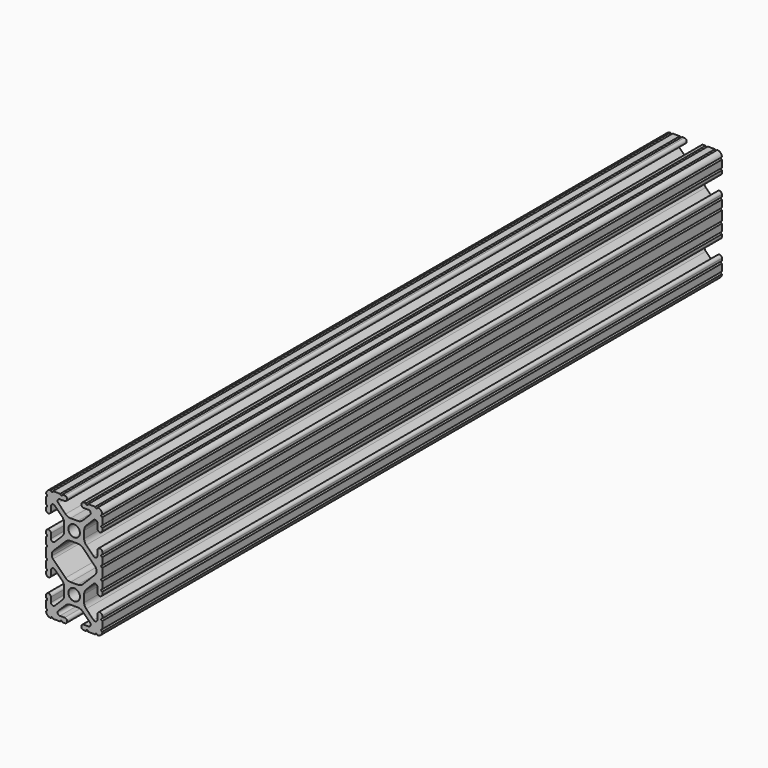
from build123d import *

# Parameters (mm, degrees)
F1_DEPTH = 350


# Not quite as in the source:
# - ends of sketch curves that miss each other by under 0.0002 mm in the source are joined


with BuildPart() as f1:
    # F0 (on Front) → F1 (new body)
    with BuildSketch(Plane.XZ):
        with BuildLine():
            ThreePointArc((-12.6999998568, 23.2791116031), (-12.1919492, 22.76475), (-12.6999998568, 22.2503883969))
            Line((-12.6999998568, 22.2503883969), (-12.7, 19.0246))
            ThreePointArc((-12.7, 19.0246), (-12.192, 18.5166), (-12.7, 18.0086))
            Line((-12.7, 18.0086), (-12.7, 17.0023028))
            ThreePointArc((-12.7, 17.0023028), (-11.5951, 15.8974028), (-10.4902, 17.0023028))
            Line((-10.4902, 17.0023028), (-10.4902, 19.1747902))
            ThreePointArc((-10.4902, 19.1747902), (-9.8630063673, 20.113451805), (-8.7557795103, 19.8932106897))
            Line((-8.7557795103, 19.8932106897), (-5.4384448, 16.5758622))
            ThreePointArc((-5.4384448, 16.5758622), (-4.7501824843, 15.5458268978), (-4.5085, 14.330807))
            Line((-4.5085, 14.330807), (-4.5085, 11.069193))
            ThreePointArc((-4.5085, 11.069193), (-4.7501824843, 9.8541731022), (-5.4384359697, 8.8241289697))
            Line((-5.4384359697, 8.8241289697), (-8.7557864, 5.5067962))
            ThreePointArc((-8.7557864, 5.5067962), (-9.8630063673, 5.286548195), (-10.4902, 6.2252098))
            Line((-10.4902, 6.2252098), (-10.4902, 8.3976972))
            ThreePointArc((-10.4902, 8.3976972), (-11.5951, 9.5025972), (-12.7, 8.3976972))
            Line((-12.7, 8.3976972), (-12.7, 7.3914))
            ThreePointArc((-12.7, 7.3914), (-12.192, 6.8834), (-12.7, 6.3754))
            Line((-12.7, 6.3754), (-12.7, 3.1496))
            ThreePointArc((-12.7, 3.1496), (-12.192, 2.6416), (-12.7, 2.1336))
            Line((-12.7, 2.1336), (-12.7, -2.1336))
            ThreePointArc((-12.7, -2.1336), (-12.192, -2.6416), (-12.7, -3.1496))
            Line((-12.7, -3.1496), (-12.7, -6.3754))
            ThreePointArc((-12.7, -6.3754), (-12.192, -6.8834), (-12.7, -7.3914))
            Line((-12.7, -7.3914), (-12.7, -8.3976972))
            ThreePointArc((-12.7, -8.3976972), (-11.5951, -9.5025972), (-10.4902, -8.3976972))
            Line((-10.4902, -8.3976972), (-10.4902, -6.2252098))
            ThreePointArc((-10.4902, -6.2252098), (-9.8630063673, -5.286548195), (-8.7557795103, -5.5067893103))
            Line((-8.7557795103, -5.5067893103), (-5.4384448, -8.8241378))
            ThreePointArc((-5.4384448, -8.8241378), (-4.7501824843, -9.8541731022), (-4.5085, -11.069193))
            Line((-4.5085, -11.069193), (-4.5085, -14.330807))
            ThreePointArc((-4.5085, -14.330807), (-4.7501824843, -15.5458268978), (-5.4384359697, -16.5758710303))
            Line((-5.4384359697, -16.5758710303), (-8.7557864, -19.8932038))
            ThreePointArc((-8.7557864, -19.8932038), (-9.8630063673, -20.113451805), (-10.4902, -19.1747902))
            Line((-10.4902, -19.1747902), (-10.4902, -17.0023028))
            ThreePointArc((-10.4902, -17.0023028), (-11.5951, -15.8974028), (-12.7, -17.0023028))
            Line((-12.7, -17.0023028), (-12.7, -18.0086))
            ThreePointArc((-12.7, -18.0086), (-12.192, -18.5166), (-12.7, -19.0246))
            Line((-12.7, -19.0246), (-12.7, -22.2504))
            ThreePointArc((-12.7, -22.2504), (-12.1919492, -22.76475), (-12.6999998568, -23.2791116031))
            ThreePointArc((-12.6999998568, -23.2791116031), (-12.0825733161, -24.7825733161), (-10.579099926, -25.4000122396))
            ThreePointArc((-10.579099926, -25.4000122396), (-10.06475, -24.8919492), (-9.5503883969, -25.3999998568))
            Line((-9.5503883969, -25.3999998568), (-6.3246, -25.4))
            ThreePointArc((-6.3246, -25.4), (-5.8166, -24.892), (-5.3086, -25.4))
            Line((-5.3086, -25.4), (-4.3023028, -25.4))
            ThreePointArc((-4.3023028, -25.4), (-3.1974028, -24.2951), (-4.3023028, -23.1902))
            Line((-4.3023028, -23.1902), (-6.4747902, -23.1902))
            ThreePointArc((-6.4747902, -23.1902), (-7.413451805, -22.5630063673), (-7.1932106897, -21.4557795103))
            Line((-7.1932106897, -21.4557795103), (-3.8758622, -18.1384448))
            ThreePointArc((-3.8758622, -18.1384448), (-2.8458268978, -17.4501824843), (-1.630807, -17.2085))
            Line((-1.630807, -17.2085), (1.630807, -17.2085))
            ThreePointArc((1.630807, -17.2085), (2.8458268978, -17.4501824843), (3.8758710303, -18.1384359697))
            Line((3.8758710303, -18.1384359697), (7.1932038, -21.4557864))
            ThreePointArc((7.1932038, -21.4557864), (7.413451805, -22.5630063673), (6.4747902, -23.1902))
            Line((6.4747902, -23.1902), (4.3023028, -23.1902))
            ThreePointArc((4.3023028, -23.1902), (3.1974028, -24.2951), (4.3023028, -25.4))
            Line((4.3023028, -25.4), (5.3086, -25.4))
            ThreePointArc((5.3086, -25.4), (5.8166, -24.892), (6.3246, -25.4))
            Line((6.3246, -25.4), (9.5504, -25.4))
            ThreePointArc((9.5504, -25.4), (10.06475, -24.8919492), (10.5791116031, -25.3999998568))
            ThreePointArc((10.5791116031, -25.3999998568), (12.0825733161, -24.7825733161), (12.7000122396, -23.279099926))
            ThreePointArc((12.7000122396, -23.279099926), (12.1919492, -22.76475), (12.6999998568, -22.2503883969))
            Line((12.6999998568, -22.2503883969), (12.7, -19.0246))
            ThreePointArc((12.7, -19.0246), (12.192, -18.5166), (12.7, -18.0086))
            Line((12.7, -18.0086), (12.7, -17.0023028))
            ThreePointArc((12.7, -17.0023028), (11.5951, -15.8974028), (10.4902, -17.0023028))
            Line((10.4902, -17.0023028), (10.4902, -19.1747902))
            ThreePointArc((10.4902, -19.1747902), (9.8630063673, -20.113451805), (8.7557795103, -19.8932106897))
            Line((8.7557795103, -19.8932106897), (5.4384448, -16.5758622))
            ThreePointArc((5.4384448, -16.5758622), (4.7501824843, -15.5458268978), (4.5085, -14.330807))
            Line((4.5085, -14.330807), (4.5085, -11.069193))
            ThreePointArc((4.5085, -11.069193), (4.7501824843, -9.8541731022), (5.4384359697, -8.8241289697))
            Line((5.4384359697, -8.8241289697), (8.7557864, -5.5067962))
            ThreePointArc((8.7557864, -5.5067962), (9.8630063673, -5.286548195), (10.4902, -6.2252098))
            Line((10.4902, -6.2252098), (10.4902, -8.3976972))
            ThreePointArc((10.4902, -8.3976972), (11.5951, -9.5025972), (12.7, -8.3976972))
            Line((12.7, -8.3976972), (12.7, -7.3914))
            ThreePointArc((12.7, -7.3914), (12.192, -6.8834), (12.7, -6.3754))
            Line((12.7, -6.3754), (12.7, -3.1496))
            ThreePointArc((12.7, -3.1496), (12.192, -2.6416), (12.7, -2.1336))
            Line((12.7, -2.1336), (12.7, 2.1336))
            ThreePointArc((12.7, 2.1336), (12.192, 2.6416), (12.7, 3.1496))
            Line((12.7, 3.1496), (12.7, 6.3754))
            ThreePointArc((12.7, 6.3754), (12.192, 6.8834), (12.7, 7.3914))
            Line((12.7, 7.3914), (12.7, 8.3976972))
            ThreePointArc((12.7, 8.3976972), (11.5951, 9.5025972), (10.4902, 8.3976972))
            Line((10.4902, 8.3976972), (10.4902, 6.2252098))
            ThreePointArc((10.4902, 6.2252098), (9.8630063673, 5.286548195), (8.7557795103, 5.5067893103))
            Line((8.7557795103, 5.5067893103), (5.4384448, 8.8241378))
            ThreePointArc((5.4384448, 8.8241378), (4.7501824843, 9.8541731022), (4.5085, 11.069193))
            Line((4.5085, 11.069193), (4.5085, 14.330807))
            ThreePointArc((4.5085, 14.330807), (4.7501824843, 15.5458268978), (5.4384359697, 16.5758710303))
            Line((5.4384359697, 16.5758710303), (8.7557864, 19.8932038))
            ThreePointArc((8.7557864, 19.8932038), (9.8630063673, 20.113451805), (10.4902, 19.1747902))
            Line((10.4902, 19.1747902), (10.4902, 17.0023028))
            ThreePointArc((10.4902, 17.0023028), (11.5951, 15.8974028), (12.7, 17.0023028))
            Line((12.7, 17.0023028), (12.7, 18.0086))
            ThreePointArc((12.7, 18.0086), (12.192, 18.5166), (12.7, 19.0246))
            Line((12.7, 19.0246), (12.7, 22.2504))
            ThreePointArc((12.7, 22.2504), (12.1919492, 22.76475), (12.6999998568, 23.2791116031))
            ThreePointArc((12.6999998568, 23.2791116031), (12.0825733161, 24.7825733161), (10.579099926, 25.4000122396))
            ThreePointArc((10.579099926, 25.4000122396), (10.06475, 24.8919492), (9.5503883969, 25.3999998568))
            Line((9.5503883969, 25.3999998568), (6.3246, 25.4))
            ThreePointArc((6.3246, 25.4), (5.8166, 24.892), (5.3086, 25.4))
            Line((5.3086, 25.4), (4.3023028, 25.4))
            ThreePointArc((4.3023028, 25.4), (3.1974028, 24.2951), (4.3023028, 23.1902))
            Line((4.3023028, 23.1902), (6.4747902, 23.1902))
            ThreePointArc((6.4747902, 23.1902), (7.413451805, 22.5630063673), (7.1932106897, 21.4557795103))
            Line((7.1932106897, 21.4557795103), (3.8758622, 18.1384448))
            ThreePointArc((3.8758622, 18.1384448), (2.8458268978, 17.4501824843), (1.630807, 17.2085))
            Line((1.630807, 17.2085), (-1.630807, 17.2085))
            ThreePointArc((-1.630807, 17.2085), (-2.8458268978, 17.4501824843), (-3.8758710303, 18.1384359697))
            Line((-3.8758710303, 18.1384359697), (-7.1932038, 21.4557864))
            ThreePointArc((-7.1932038, 21.4557864), (-7.413451805, 22.5630063673), (-6.4747902, 23.1902))
            Line((-6.4747902, 23.1902), (-4.3023028, 23.1902))
            ThreePointArc((-4.3023028, 23.1902), (-3.1974028, 24.2951), (-4.3023028, 25.4))
            Line((-4.3023028, 25.4), (-5.3086, 25.4))
            ThreePointArc((-5.3086, 25.4), (-5.8166, 24.892), (-6.3246, 25.4))
            Line((-6.3246, 25.4), (-9.5504, 25.4))
            ThreePointArc((-9.5504, 25.4), (-10.06475, 24.8919492), (-10.5791116031, 25.3999998568))
            ThreePointArc((-10.5791116031, 25.3999998568), (-12.0825733161, 24.7825733161), (-12.6999998568, 23.2791116031))
        make_face()
        with BuildLine():
            ThreePointArc((-2.6035, -12.7), (0, -10.0965), (2.6035, -12.7))
            ThreePointArc((2.6035, -12.7), (0, -15.3035), (-2.6035, -12.7))
        make_face(mode=Mode.SUBTRACT)
        with BuildLine():
            ThreePointArc((-10.033, 0.45212), (-9.9131254878, 1.0547698693), (-9.571751759, 1.565671759))
            Line((-9.571751759, 1.565671759), (-3.8758622, 7.2615552))
            ThreePointArc((-3.8758622, 7.2615552), (-2.8458268978, 7.9498175157), (-1.630807, 8.1915))
            Line((-1.630807, 8.1915), (1.630807, 8.1915))
            ThreePointArc((1.630807, 8.1915), (2.8458268978, 7.9498175157), (3.8758710303, 7.2615640303))
            Line((3.8758710303, 7.2615640303), (9.5717614, 1.5656814))
            ThreePointArc((9.5717614, 1.5656814), (9.9131254878, 1.0547698693), (10.033, 0.45212))
            Line((10.033, 0.45212), (10.033, -0.45212))
            ThreePointArc((10.033, -0.45212), (9.9131254878, -1.0547698693), (9.571751759, -1.565671759))
            Line((9.571751759, -1.565671759), (3.8758622, -7.2615552))
            ThreePointArc((3.8758622, -7.2615552), (2.8458268978, -7.9498175157), (1.630807, -8.1915))
            Line((1.630807, -8.1915), (-1.630807, -8.1915))
            ThreePointArc((-1.630807, -8.1915), (-2.8458268978, -7.9498175157), (-3.8758710303, -7.2615640303))
            Line((-3.8758710303, -7.2615640303), (-9.5717614, -1.5656814))
            ThreePointArc((-9.5717614, -1.5656814), (-9.9131254878, -1.0547698693), (-10.033, -0.45212))
            Line((-10.033, -0.45212), (-10.033, 0.45212))
        make_face(mode=Mode.SUBTRACT)
        with BuildLine():
            ThreePointArc((-2.6035, 12.7), (0, 15.3035), (2.6035, 12.7))
            ThreePointArc((2.6035, 12.7), (0, 10.0965), (-2.6035, 12.7))
        make_face(mode=Mode.SUBTRACT)
    extrude(amount=F1_DEPTH)


solid = f1.part
